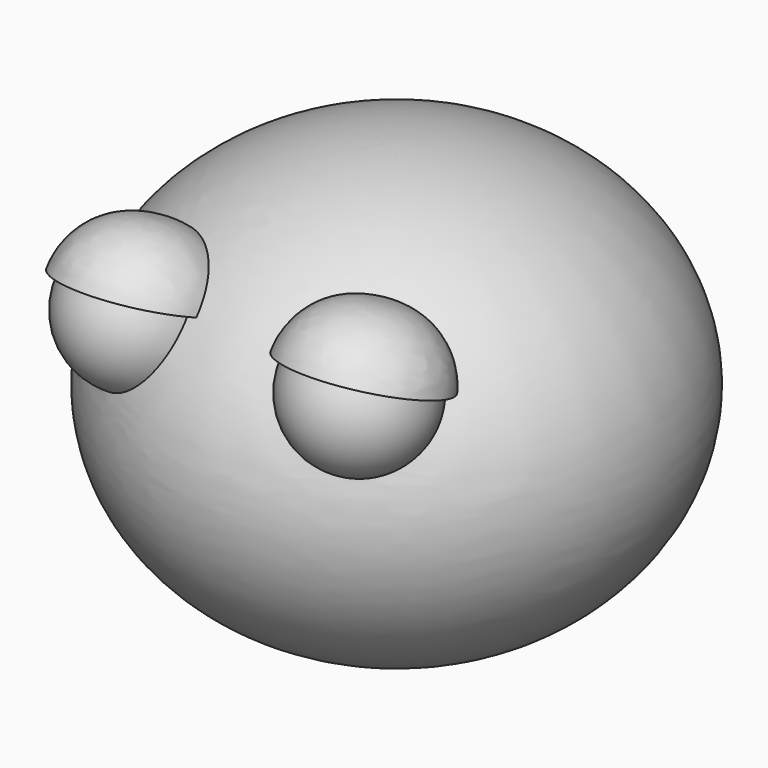
from build123d import *


with BuildPart() as f1:
    # F0 (on Front) → F1 (revolve)
    with BuildSketch(Plane.XZ):
        with BuildLine():
            Line((0, -28.5), (0, 28.5))
            add(Edge.make_bspline(
                [(0, 28.5), (-34, 28.5), (-34, 0), (-34, -28.5), (0, -28.5)],
                knots=[4.7123889804, 4.7123889804, 4.7123889804, 6.2831853072, 6.2831853072, 7.853981634, 7.853981634, 7.853981634], degree=2, weights=[1, 0.7071067812, 1, 0.7071067812, 1]))
        make_face()
    revolve(axis=Axis((0, 0, 19.9207719415), (0, 0, 1)))

    # F3 (on offset) → F4 (revolve)
    with BuildSketch(Plane.XZ.offset(25)):
        with BuildLine():
            Line((-15, 5), (-15, 23))
            ThreePointArc((-15, 23), (-24, 14), (-15, 5))
        make_face()
    revolve(axis=Axis((-15, -25, 22.264403075), (0, 0, 1)))

    # F3 (on offset) → F5 (revolve)
    with BuildSketch(Plane.XZ.offset(25)):
        with BuildLine():
            Line((15, 5), (15, 23))
            ThreePointArc((15, 23), (6, 14), (15, 5))
        make_face()
    revolve(axis=Axis((15, -25, 22.264403075), (0, 0, 1)))

    # F7 (on face) → F8 (revolve)
    with BuildSketch(Plane(origin=(0, -26.5750688068, 9.6725340192), x_dir=(1, 0, 0), z_dir=(0, -0.9396926208, 0.3420201433))):
        with BuildLine():
            ThreePointArc((-15, 4.7772144899), (-10.1387464853, 6.4850377946), (-4.9945187539, 6.7772144899))
            ThreePointArc((-4.9945187539, 6.7772144899), (-8.3920707363, 12.7848000949), (-15, 14.7772144899))
            Line((-15, 14.7772144899), (-15, 4.7772144899))
        make_face()
    revolve(axis=Axis((-15, -22.0597733627, 22.0782062941), (0, 0.3420201433, 0.9396926208)))

    # F9: F1 across plane


with BuildPart() as f1_1:
    add(f1.part)
    add(f1.part.mirror(Plane.YZ))


solid = f1_1.part
